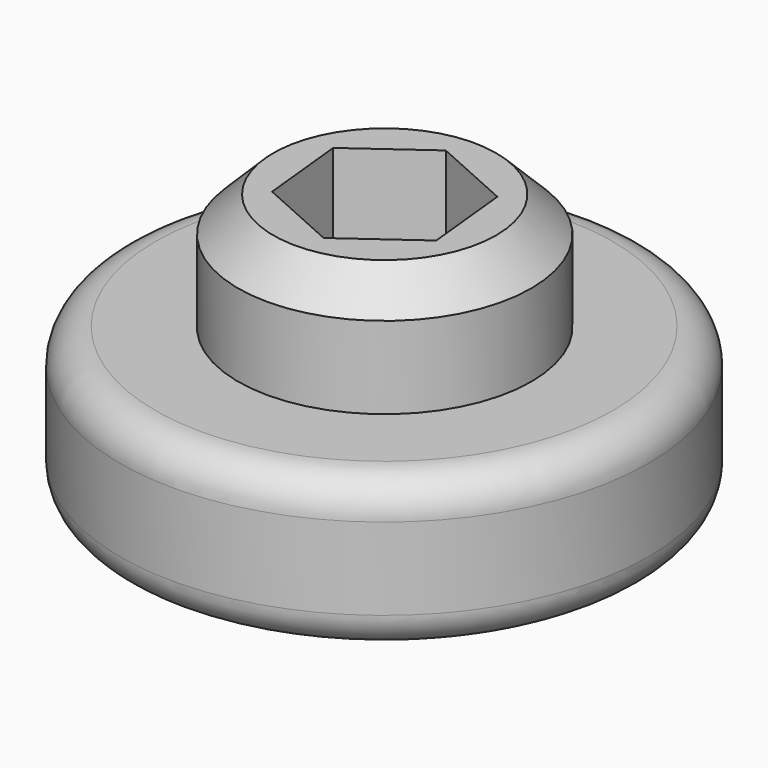
from build123d import *

# Parameters (mm, degrees)
F1_R     = 12.5
F2_DEPTH = 13
F0_R     = 22.5
F3_DEPTH = 10
F5_R     = 3
F6_SIZE  = 3
F8_DEPTH = 9


# Not quite as in the source:
# - the program builds the solid bodies; features that only make, move or delete a surface that nothing else refers to are left out


with BuildPart() as f2:
    # F1 (on Top) → F2 (new body)
    with BuildSketch(Plane.XY):
        with Locations((-37.169251591, 37.6385599375)):
            Circle(F1_R)
    extrude(amount=F2_DEPTH)

    # F3 (add): a face of the model
    f3_faces = [f2.faces().sort_by_distance(p)[0] for p in [
        (-37.169251591, 37.6385599375, 13),
    ]]


with BuildPart() as f2b:
    # F0 (on Top) → F2, piece 2 (new body)
    with BuildSketch(Plane.XY):
        with Locations((-37.3275603359, 37.7723030881)):
            Circle(F0_R)
    extrude(amount=F2_DEPTH)


with BuildPart() as f2_1:
    add(f2.part)

    add(f2b.part)  # F3 merges F2b
    extrude(f3_faces, amount=F3_DEPTH)

    # F5
    f5_edges = [f2_1.edges().sort_by_distance(p)[0] for p in [
        (-59.82756, 37.772303, 13),
        (-59.82756, 37.772303, 0),
    ]]
    fillet(f5_edges, radius=F5_R)

    # F6
    f6_edges = [f2_1.edges().sort_by_distance(p)[0] for p in [
        (-49.669252, 37.63856, 23),
    ]]
    chamfer(f6_edges, length=F6_SIZE)

    # F4 (on face) → F8 (cut)
    with BuildSketch(Plane.XY.offset(23)):
        Polygon((-36.4021524321, 30.1723097264), (-30.3197396578, 34.5697621907), (-31.0868388166, 42.0360124018), (-37.9363507498, 45.1048101485), (-44.0187635242, 40.7073576842), (-43.2516643653, 33.2411074732), align=None)
    extrude(amount=-F8_DEPTH, mode=Mode.SUBTRACT)


solid = f2_1.part
